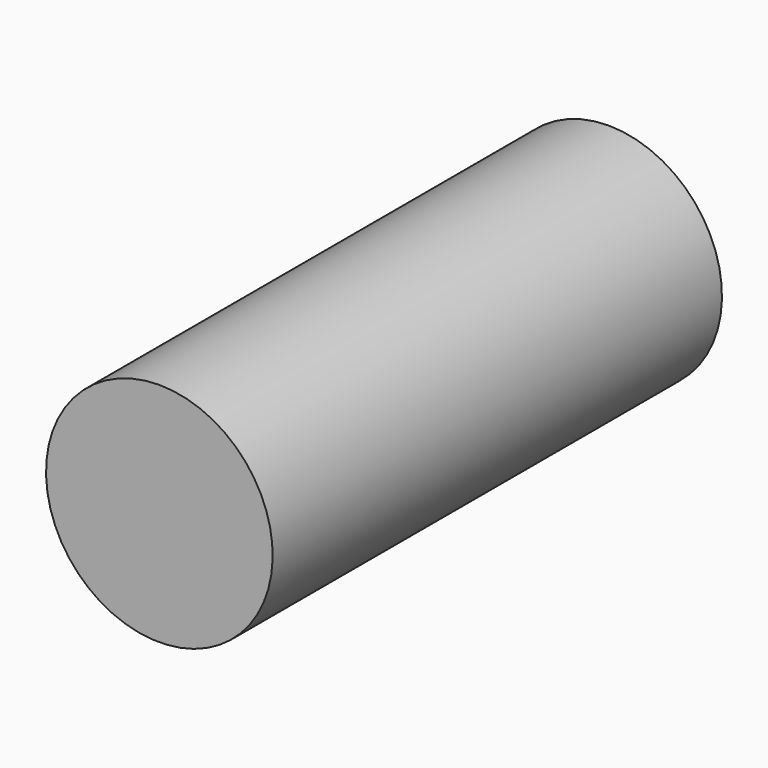
from build123d import *

# Parameters (mm, degrees)
F1_W = 323.4012946486
F1_H = 65.2434378862


# Not quite as in the source:
# - a feature names something its author has since deleted; it is built from what else it names


with BuildPart() as f2:
    # F1 (on face) → F2 (revolve)
    with BuildSketch(Plane.YZ):
        with Locations((89.398752898, 47.5624650717)):
            Rectangle(F1_W, F1_H)
    revolve(axis=Axis((0, 89.398752898, 14.9407461286), (0, 1, 0)))


solid = f2.part
